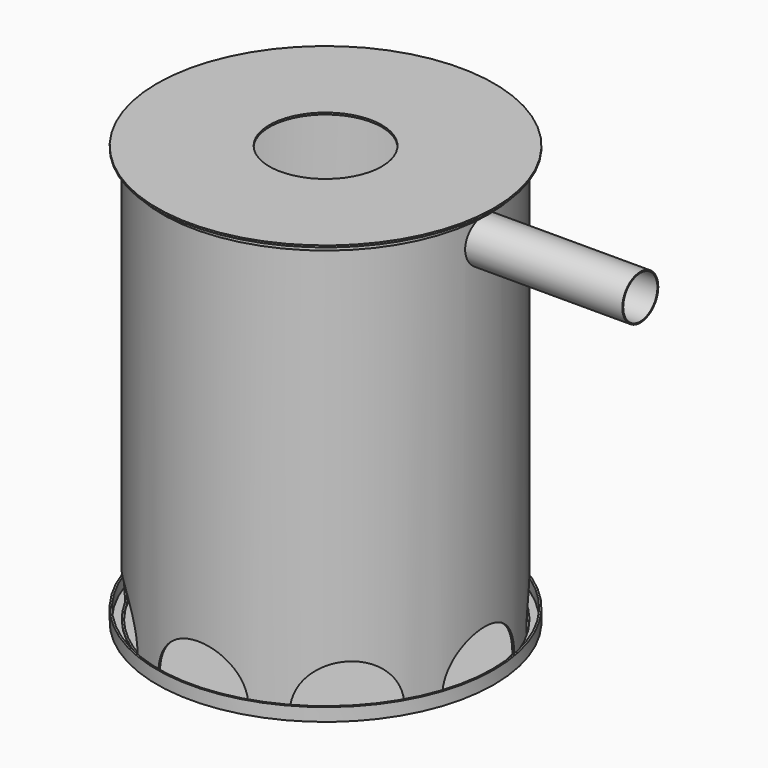
from build123d import *

# Parameters (mm, degrees)
F2_R      = 5
F3_DEPTH  = 1.6
F4_R      = 20
F5_DEPTH  = 280
F6_R      = 19
F7_DEPTH  = 280.0010001
F9_DEPTH  = 150
F10_COUNT = 8
F12_R     = 5
F13_DEPTH = 128
F14_COUNT = 4
F16_R     = 140
F17_DEPTH = 52
F18_R     = 150
F19_DEPTH = 1.6
F21_R     = 50
F22_DEPTH = 2
F23_R     = 150
F24_DEPTH = 1.6
F25_R     = 150
F25_R_2   = 148.4
F26_DEPTH = 10
F20_R     = 145.1
F20_R_2   = 143.5
F27_DEPTH = 5


# Not quite as in the source:
# - a feature names something its author has since deleted; it is built from what else it names


with BuildPart() as f1:
    # F0 (on Front) → F1 (revolve)
    with BuildSketch(Plane.XZ):
        Polygon((140, 50.4), (140, 0), (141.6, 0), (141.6, 370), (140, 370), (140, 52), align=None)
        Polygon((0, 50.4), (140, 50.4), (140, 52), (115, 52), (113.4, 52), (0, 52), align=None)
        Polygon((113.4, 52), (115, 52), (115, 192.5823523748), (51.6, 268.1395301453), (51.6, 318), (50, 318), (50, 267.5571777705), (113.4, 192), align=None)
    revolve(axis=Axis((0, 0, 185.5), (0, 0, 1)))

    # F2 (on face) → F3 (cut, through all)
    with BuildSketch(Plane.XY.offset(52)):
        Circle(F2_R)
        with Locations((20, 0)):
            Circle(F2_R)
        with Locations((10, 17.3205080757)):
            Circle(F2_R)
        with Locations((-10, 17.3205080757)):
            Circle(F2_R)
        with Locations((-20, 0)):
            Circle(F2_R)
        with Locations((40, 0)):
            Circle(F2_R)
        with Locations((34.6410161514, 20)):
            Circle(F2_R)
        with Locations((20, 34.6410161514)):
            Circle(F2_R)
        with Locations((0, 40)):
            Circle(F2_R)
        with Locations((-20, 34.6410161514)):
            Circle(F2_R)
        with Locations((-34.6410161514, 20)):
            Circle(F2_R)
        with Locations((-40, 0)):
            Circle(F2_R)
        with Locations((-34.6410161514, -20)):
            Circle(F2_R)
        with Locations((60, 0)):
            Circle(F2_R)
        with Locations((80, 0)):
            Circle(F2_R)
        with Locations((57.0633909777, 18.5410196625)):
            Circle(F2_R)
        with Locations((48.5410196625, 35.2671151375)):
            Circle(F2_R)
        with Locations((35.2671151375, 48.5410196625)):
            Circle(F2_R)
        with Locations((18.5410196625, 57.0633909777)):
            Circle(F2_R)
        with Locations((0, 60)):
            Circle(F2_R)
        with Locations((-18.5410196625, 57.0633909777)):
            Circle(F2_R)
        with Locations((-35.2671151375, 48.5410196625)):
            Circle(F2_R)
        with Locations((-48.5410196625, 35.2671151375)):
            Circle(F2_R)
        with Locations((-57.0633909777, 18.5410196625)):
            Circle(F2_R)
        with Locations((-60, 0)):
            Circle(F2_R)
        with Locations((-57.0633909777, -18.5410196625)):
            Circle(F2_R)
        with Locations((-48.5410196625, -35.2671151375)):
            Circle(F2_R)
        with Locations((-35.2671151375, -48.5410196625)):
            Circle(F2_R)
        with Locations((-18.5410196625, -57.0633909777)):
            Circle(F2_R)
        with Locations((0, -60)):
            Circle(F2_R)
        with Locations((18.5410196625, -57.0633909777)):
            Circle(F2_R)
        with Locations((35.2671151375, -48.5410196625)):
            Circle(F2_R)
        with Locations((48.5410196625, -35.2671151375)):
            Circle(F2_R)
        with Locations((57.0633909777, -18.5410196625)):
            Circle(F2_R)
        with Locations((-20, -34.6410161514)):
            Circle(F2_R)
        with Locations((0, -40)):
            Circle(F2_R)
        with Locations((20, -34.6410161514)):
            Circle(F2_R)
        with Locations((34.6410161514, -20)):
            Circle(F2_R)
        with Locations((77.9942329745, 17.8016747165)):
            Circle(F2_R)
        with Locations((72.0775094322, 34.7106991294)):
            Circle(F2_R)
        with Locations((62.5465185974, 49.8791841487)):
            Circle(F2_R)
        with Locations((49.8791841487, 62.5465185974)):
            Circle(F2_R)
        with Locations((34.7106991294, 72.0775094322)):
            Circle(F2_R)
        with Locations((17.8016747165, 77.9942329745)):
            Circle(F2_R)
        with Locations((0, 80)):
            Circle(F2_R)
        with Locations((-17.8016747165, 77.9942329745)):
            Circle(F2_R)
        with Locations((-34.7106991294, 72.0775094322)):
            Circle(F2_R)
        with Locations((-49.8791841487, 62.5465185974)):
            Circle(F2_R)
        with Locations((-62.5465185974, 49.8791841487)):
            Circle(F2_R)
        with Locations((-72.0775094322, 34.7106991294)):
            Circle(F2_R)
        with Locations((-77.9942329745, 17.8016747165)):
            Circle(F2_R)
        with Locations((-80, 0)):
            Circle(F2_R)
        with Locations((-77.9942329745, -17.8016747165)):
            Circle(F2_R)
        with Locations((-72.0775094322, -34.7106991294)):
            Circle(F2_R)
        with Locations((-62.5465185974, -49.8791841487)):
            Circle(F2_R)
        with Locations((-49.8791841487, -62.5465185974)):
            Circle(F2_R)
        with Locations((-34.7106991294, -72.0775094322)):
            Circle(F2_R)
        with Locations((-17.8016747165, -77.9942329745)):
            Circle(F2_R)
        with Locations((0, -80)):
            Circle(F2_R)
        with Locations((17.8016747165, -77.9942329745)):
            Circle(F2_R)
        with Locations((34.7106991294, -72.0775094322)):
            Circle(F2_R)
        with Locations((49.8791841487, -62.5465185974)):
            Circle(F2_R)
        with Locations((62.5465185974, -49.8791841487)):
            Circle(F2_R)
        with Locations((72.0775094322, -34.7106991294)):
            Circle(F2_R)
        with Locations((77.9942329745, -17.8016747165)):
            Circle(F2_R)
        with Locations((-10, -17.3205080757)):
            Circle(F2_R)
        with Locations((10, -17.3205080757)):
            Circle(F2_R)
    extrude(amount=-F3_DEPTH, mode=Mode.SUBTRACT)

    # F4 (on Right) → F5 (join)
    with BuildSketch(Plane.YZ):
        with Locations((0, 344)):
            Circle(F4_R)
    extrude(amount=F5_DEPTH)

    # F6 (on face) → F7 (cut, through all)
    with BuildSketch(Plane(origin=(0, 0, 0), x_dir=(0, -1, 0), z_dir=(-1, 0, 0))):
        with Locations((0, 344)):
            Circle(F6_R)
    extrude(amount=-F7_DEPTH, mode=Mode.SUBTRACT)


with BuildPart() as f9:
    # F8 (on Front) → F9 (new body)
    with BuildSketch(Plane.XZ):
        with BuildLine():
            Line((-40, 1), (0, 1))
            Line((0, 1), (40, 1))
            ThreePointArc((40, 1), (0, 41), (-40, 1))
        make_face()
    extrude(amount=F9_DEPTH)


with BuildPart() as f10_1:
    # F10: instance of F9
    add(f9.part.rotate(Axis((0, 0, 185.5), (0, 0, 1)), 1 * 360 / F10_COUNT))


with BuildPart() as f10_2:
    # F10: instance of F9
    add(f9.part.rotate(Axis((0, 0, 185.5), (0, 0, 1)), 2 * 360 / F10_COUNT))


with BuildPart() as f10_3:
    # F10: instance of F9
    add(f9.part.rotate(Axis((0, 0, 185.5), (0, 0, 1)), 3 * 360 / F10_COUNT))


with BuildPart() as f10_4:
    # F10: instance of F9
    add(f9.part.rotate(Axis((0, 0, 185.5), (0, 0, 1)), 4 * 360 / F10_COUNT))


with BuildPart() as f10_5:
    # F10: instance of F9
    add(f9.part.rotate(Axis((0, 0, 185.5), (0, 0, 1)), 5 * 360 / F10_COUNT))


with BuildPart() as f10_6:
    # F10: instance of F9
    add(f9.part.rotate(Axis((0, 0, 185.5), (0, 0, 1)), 6 * 360 / F10_COUNT))


with BuildPart() as f10_7:
    # F10: instance of F9
    add(f9.part.rotate(Axis((0, 0, 185.5), (0, 0, 1)), 7 * 360 / F10_COUNT))


with BuildPart() as f1_1:
    add(f1.part)

    # F11: cut F9, F10_1, F10_2, F10_3, F10_4, F10_5, F10_6, F10_7
    add(f9.part, mode=Mode.SUBTRACT)
    add(f10_1.part, mode=Mode.SUBTRACT)
    add(f10_2.part, mode=Mode.SUBTRACT)
    add(f10_3.part, mode=Mode.SUBTRACT)
    add(f10_4.part, mode=Mode.SUBTRACT)
    add(f10_5.part, mode=Mode.SUBTRACT)
    add(f10_6.part, mode=Mode.SUBTRACT)
    add(f10_7.part, mode=Mode.SUBTRACT)


with BuildPart() as f13:
    # F12 (on Front) → F13 (new body)
    with BuildSketch(Plane.XZ):
        with Locations((0, 151)):
            Circle(F12_R)
    extrude(amount=F13_DEPTH)


with BuildPart() as f14_1:
    # F14: instance of F13
    add(f13.part.rotate(Axis((0, 0, 185.5), (0, 0, 1)), 1 * 360 / F14_COUNT))


with BuildPart() as f14_2:
    # F14: instance of F13
    add(f13.part.rotate(Axis((0, 0, 185.5), (0, 0, 1)), 2 * 360 / F14_COUNT))


with BuildPart() as f14_3:
    # F14: instance of F13
    add(f13.part.rotate(Axis((0, 0, 185.5), (0, 0, 1)), 3 * 360 / F14_COUNT))


with BuildPart() as f1_2:
    add(f1_1.part)

    # F15: cut F14_2, F14_3, F14_1, F13
    add(f14_2.part, mode=Mode.SUBTRACT)
    add(f14_3.part, mode=Mode.SUBTRACT)
    add(f14_1.part, mode=Mode.SUBTRACT)
    add(f13.part, mode=Mode.SUBTRACT)

    # F16 (on face) → F17 (cut, through all)
    with BuildSketch(Plane.XY.offset(370)):
        Circle(F16_R)
    extrude(amount=-F17_DEPTH, mode=Mode.SUBTRACT)


with BuildPart() as f19:
    # F18 (on face) → F19 (new body)
    with BuildSketch(Plane.XY.offset(370)):
        Circle(F18_R)
    extrude(amount=F19_DEPTH)

    # F21 (on face) → F22 (cut)
    with BuildSketch(Plane.XY.offset(371.6)):
        Circle(F21_R)
    extrude(amount=-F22_DEPTH, mode=Mode.SUBTRACT)


with BuildPart() as f24:
    # F23 (on face) → F24 (new body)
    with BuildSketch(Plane(origin=(0, 0, 0), x_dir=(1, 0, 0), z_dir=(0, 0, -1))):
        Circle(F23_R)
    extrude(amount=F24_DEPTH)

    # F25 (on face) → F26 (join)
    with BuildSketch(Plane.XY):
        Circle(F25_R)
        Circle(F25_R_2, mode=Mode.SUBTRACT)
    extrude(amount=F26_DEPTH)


with BuildPart() as f27:
    # F20 (on face) → F27 (new body)
    with BuildSketch(Plane(origin=(0, 0, 370), x_dir=(1, 0, 0), z_dir=(0, 0, -1))):
        Circle(F20_R)
        Circle(F20_R_2, mode=Mode.SUBTRACT)
    extrude(amount=F27_DEPTH)


solid = Compound([f1_2.part, f19.part, f24.part, f27.part])
